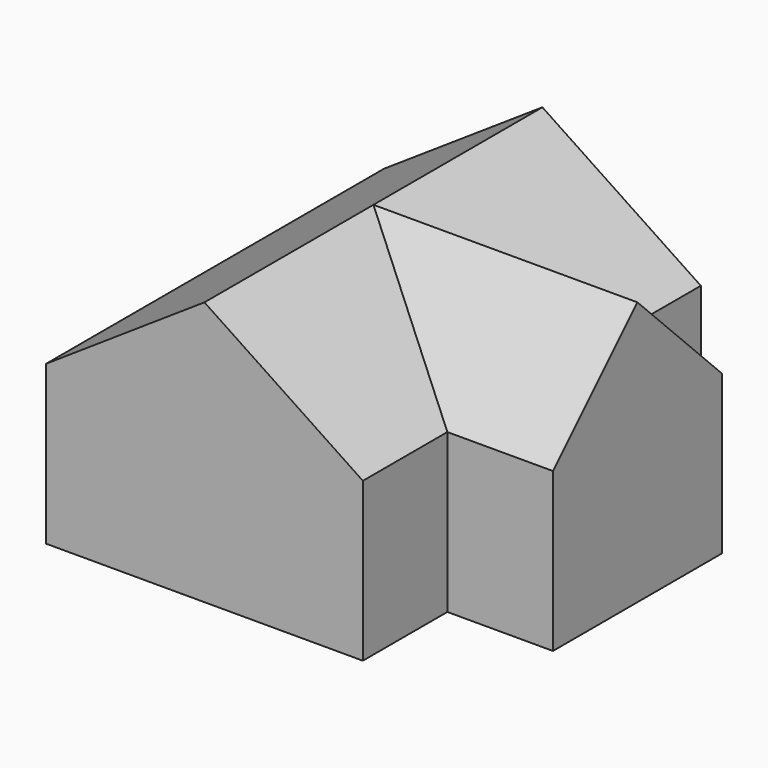
from build123d import *

# Parameters (mm, degrees)
F1_DEPTH = 50.8
F2_W     = 25.4
F2_H     = 31.75
F3_DEPTH = 12.7
F5_DEPTH = 50.8
F7_DEPTH = 12.7
F8_DEPTH = 31.75


with BuildPart() as f1:
    # F0 (on Front) → F1 (new body)
    with BuildSketch(Plane.XZ):
        Polygon((0, 19.05), (0, 0), (38.1, 0), (38.1, 19.05), (38.1, 31.75), (19.05, 31.75), align=None)
    extrude(amount=F1_DEPTH)

    # F2 (on face) → F3 (join)
    with BuildSketch(Plane.YZ.offset(38.1)):
        with Locations((-25.4, 15.875)):
            Rectangle(F2_W, F2_H)
    extrude(amount=F3_DEPTH)

    # F4 (on face) → F5 (cut)
    with BuildSketch(Plane.XZ.offset(50.8)):
        Polygon((38.1, 31.75), (19.05, 31.75), (38.1, 19.05), align=None)
    extrude(amount=-F5_DEPTH, mode=Mode.SUBTRACT)

    # F6 (on face) → F7 (cut)
    with BuildSketch(Plane.YZ.offset(50.8)):
        Polygon((-38.1, 31.75), (-38.1, 19.05), (-25.4, 31.75), align=None)
        Polygon((-12.7, 31.75), (-25.4, 31.75), (-12.7, 19.05), align=None)
    extrude(amount=-F7_DEPTH, mode=Mode.SUBTRACT)

    # F8 (add): a face of the model
    f8_faces = [f1.faces().sort_by_distance(p)[0] for p in [
        (50.8, -25.4, 12.9645833333),
    ]]
    extrude(f8_faces, amount=-F8_DEPTH)


solid = f1.part
